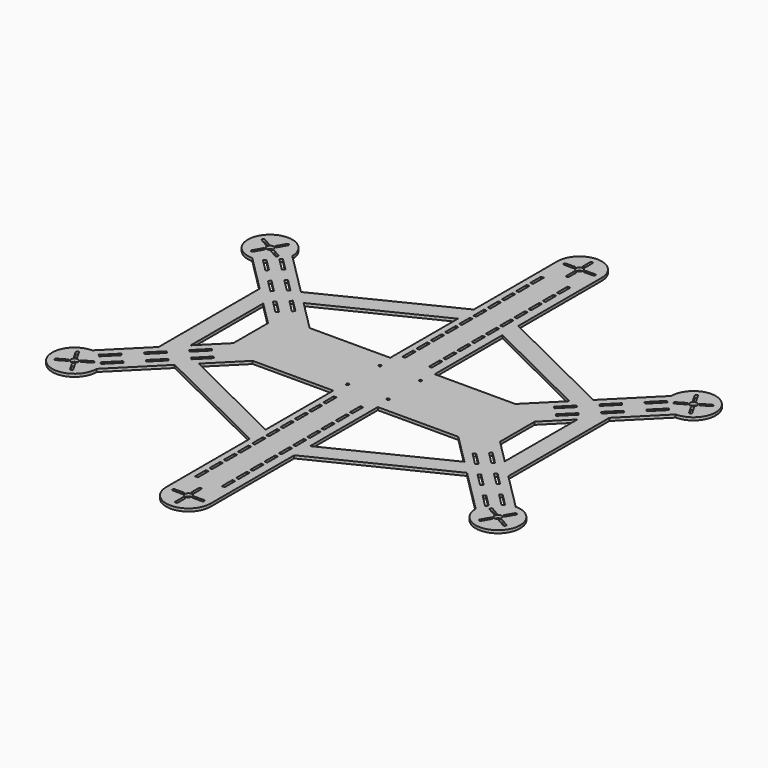
from build123d import *

# Parameters (mm, degrees)
F1_DEPTH  = 3.175
F2_W      = 3.175
F2_H      = 15
F3_DEPTH  = 25
F5_DEPTH  = 25
F6_DEPTH  = 3.175
F7_R      = 1.5
F8_DEPTH  = 25
F9_R      = 4
F9_W      = 3
F9_H      = 10
F9_W_2    = 10
F9_H_2    = 3
F10_DEPTH = 25


with BuildPart() as f1:
    # F0 (on Top) → F1 (new body)
    with BuildSketch(Plane.XY):
        with BuildLine():
            Line((-25, 275), (25, 275))
            ThreePointArc((25, 275), (0, 300), (-25, 275))
        make_face()
        with BuildLine():
            Line((25, 157.5), (25, 275))
            ThreePointArc((25, 275), (0, 250), (-25, 275))
            Line((-25, 275), (-25, 157.5))
            Line((-25, 157.5), (-25, 135.2001601372))
            Line((-25, 135.2001601372), (-25, 40))
            Line((-25, 40), (25, 40))
            Line((25, 40), (25, 135.2001601372))
            Line((25, 135.2001601372), (25, 157.5))
        make_face()
        with BuildLine():
            ThreePointArc((-25, 275), (0, 250), (25, 275))
            Line((25, 275), (-25, 275))
        make_face()
        Polygon((164.4069860407, 88.75), (25, 157.5), (25, 135.2001601372), (149.4723277158, 73.8153416751), align=None)
        Polygon((-25, 135.2001601372), (-25, 157.5), (-164.4069860407, 88.75), (-149.4723277158, 73.8153416751), align=None)
        with BuildLine():
            Line((213.1569860407, 137.5), (164.4069860407, 88.75))
            Line((164.4069860407, 88.75), (149.4723277158, 73.8153416751))
            Line((149.4723277158, 73.8153416751), (115.6569860407, 40))
            Line((115.6569860407, 40), (150, 40))
            Line((150, 40), (150, 24.3430139593))
            Line((150, 24.3430139593), (164.5977680896, 38.9407820489))
            Line((164.5977680896, 38.9407820489), (176.670305631, 51.0133195903))
            Line((176.670305631, 51.0133195903), (188.7428431724, 63.0858571317))
            Line((188.7428431724, 63.0858571317), (196.670305631, 71.0133195903))
            Line((196.670305631, 71.0133195903), (238.1569860407, 112.5))
            ThreePointArc((238.1569860407, 112.5), (220.4793165111, 119.8223304703), (213.1569860407, 137.5))
        make_face()
        with BuildLine():
            Line((-149.4723277158, 73.8153416751), (-164.4069860407, 88.75))
            Line((-164.4069860407, 88.75), (-213.1569860407, 137.5))
            ThreePointArc((-213.1569860407, 137.5), (-220.4793165111, 119.8223304703), (-238.1569860407, 112.5))
            Line((-238.1569860407, 112.5), (-196.670305631, 71.0133195903))
            Line((-196.670305631, 71.0133195903), (-188.7428431724, 63.0858571317))
            Line((-188.7428431724, 63.0858571317), (-176.670305631, 51.0133195903))
            Line((-176.670305631, 51.0133195903), (-164.5977680896, 38.9407820489))
            Line((-164.5977680896, 38.9407820489), (-150, 24.3430139593))
            Line((-150, 24.3430139593), (-150, 40))
            Line((-150, 40), (-115.6569860407, 40))
            Line((-115.6569860407, 40), (-149.4723277158, 73.8153416751))
        make_face()
        Polygon((115.6569860407, 40), (25, 40), (-25, 40), (-115.6569860407, 40), (-150, 40), (-150, 24.3430139593), (-150, -24.3430139593), (-150, -40), (-115.6569860407, -40), (-25, -40), (25, -40), (115.6569860407, -40), (150, -40), (150, -24.3430139593), (150, 24.3430139593), (150, 40), align=None)
        with BuildLine():
            ThreePointArc((263.1569860407, 137.5), (238.1569860407, 162.5), (213.1569860407, 137.5))
            ThreePointArc((213.1569860407, 137.5), (220.4793165111, 119.8223304703), (238.1569860407, 112.5))
            Line((238.1569860407, 112.5), (263.1569860407, 137.5))
        make_face()
        with BuildLine():
            ThreePointArc((-238.1569860407, 112.5), (-220.4793165111, 119.8223304703), (-213.1569860407, 137.5))
            ThreePointArc((-213.1569860407, 137.5), (-238.1569860407, 162.5), (-263.1569860407, 137.5))
            Line((-263.1569860407, 137.5), (-238.1569860407, 112.5))
        make_face()
        with BuildLine():
            ThreePointArc((238.1569860407, 112.5), (255.8346555704, 119.8223304703), (263.1569860407, 137.5))
            Line((263.1569860407, 137.5), (238.1569860407, 112.5))
        make_face()
        with BuildLine():
            Line((-238.1569860407, 112.5), (-263.1569860407, 137.5))
            ThreePointArc((-263.1569860407, 137.5), (-255.8346555704, 119.8223304703), (-238.1569860407, 112.5))
        make_face()
        Polygon((196.670305631, -71.0133195903), (196.670305631, 71.0133195903), (188.7428431724, 63.0858571317), (176.670305631, 51.0133195903), (176.670305631, -51.0133195903), align=None)
        Polygon((-188.7428431724, 63.0858571317), (-196.670305631, 71.0133195903), (-196.670305631, -71.0133195903), (-188.7428431724, -63.0858571317), (-176.670305631, -51.0133195903), (-176.670305631, 51.0133195903), align=None)
        with BuildLine():
            Line((238.1569860407, -112.5), (196.670305631, -71.0133195903))
            Line((196.670305631, -71.0133195903), (176.670305631, -51.0133195903))
            Line((176.670305631, -51.0133195903), (150, -24.3430139593))
            Line((150, -24.3430139593), (150, -40))
            Line((150, -40), (115.6569860407, -40))
            Line((115.6569860407, -40), (149.4723277158, -73.8153416751))
            Line((149.4723277158, -73.8153416751), (164.4069860407, -88.75))
            Line((164.4069860407, -88.75), (213.1569860407, -137.5))
            ThreePointArc((213.1569860407, -137.5), (220.4793165111, -119.8223304703), (238.1569860407, -112.5))
        make_face()
        with BuildLine():
            Line((-188.7428431724, -63.0858571317), (-196.670305631, -71.0133195903))
            Line((-196.670305631, -71.0133195903), (-238.1569860407, -112.5))
            ThreePointArc((-238.1569860407, -112.5), (-220.4793165111, -119.8223304703), (-213.1569860407, -137.5))
            Line((-213.1569860407, -137.5), (-164.4069860407, -88.75))
            Line((-164.4069860407, -88.75), (-149.4723277158, -73.8153416751))
            Line((-149.4723277158, -73.8153416751), (-115.6569860407, -40))
            Line((-115.6569860407, -40), (-150, -40))
            Line((-150, -40), (-150, -24.3430139593))
            Line((-150, -24.3430139593), (-164.5977680896, -38.9407820489))
            Line((-164.5977680896, -38.9407820489), (-176.670305631, -51.0133195903))
            Line((-176.670305631, -51.0133195903), (-188.7428431724, -63.0858571317))
        make_face()
        with BuildLine():
            Line((263.1569860407, -137.5), (238.1569860407, -112.5))
            ThreePointArc((238.1569860407, -112.5), (220.4793165111, -119.8223304703), (213.1569860407, -137.5))
            ThreePointArc((213.1569860407, -137.5), (238.1569860407, -162.5), (263.1569860407, -137.5))
        make_face()
        with BuildLine():
            ThreePointArc((263.1569860407, -137.5), (255.8346555704, -119.8223304703), (238.1569860407, -112.5))
            Line((238.1569860407, -112.5), (263.1569860407, -137.5))
        make_face()
        with BuildLine():
            Line((-263.1569860407, -137.5), (-238.1569860407, -112.5))
            ThreePointArc((-238.1569860407, -112.5), (-255.8346555704, -119.8223304703), (-263.1569860407, -137.5))
        make_face()
        with BuildLine():
            ThreePointArc((-213.1569860407, -137.5), (-220.4793165111, -119.8223304703), (-238.1569860407, -112.5))
            Line((-238.1569860407, -112.5), (-263.1569860407, -137.5))
            ThreePointArc((-263.1569860407, -137.5), (-238.1569860407, -162.5), (-213.1569860407, -137.5))
        make_face()
        Polygon((25, -157.5), (164.4069860407, -88.75), (149.4723277158, -73.8153416751), (25, -135.2001601372), align=None)
        Polygon((-149.4723277158, -73.8153416751), (-164.4069860407, -88.75), (-25, -157.5), (-25, -135.2001601372), align=None)
        with BuildLine():
            Line((25, -135.2001601372), (25, -40))
            Line((25, -40), (-25, -40))
            Line((-25, -40), (-25, -135.2001601372))
            Line((-25, -135.2001601372), (-25, -157.5))
            Line((-25, -157.5), (-25, -275))
            ThreePointArc((-25, -275), (0, -250), (25, -275))
            Line((25, -275), (25, -157.5))
            Line((25, -157.5), (25, -135.2001601372))
        make_face()
        with BuildLine():
            ThreePointArc((-25, -275), (0, -300), (25, -275))
            ThreePointArc((25, -275), (0, -250), (-25, -275))
        make_face()
    extrude(amount=F1_DEPTH)

    # F2 (on face) → F3 (cut)
    with BuildSketch(Plane.XY.offset(3.175)):
        with Locations((-16.3512844592, 235.6171465556)):
            Rectangle(F2_W, F2_H)
        with Locations((13.6487155408, 235.6171465556)):
            Rectangle(F2_W, F2_H)
        with Locations((-16.3512844592, 215.6171465556)):
            Rectangle(F2_W, F2_H)
        with Locations((13.6487155408, 215.6171465556)):
            Rectangle(F2_W, F2_H)
        with Locations((-16.3512844592, 195.6171465556)):
            Rectangle(F2_W, F2_H)
        with Locations((13.6487155408, 195.6171465556)):
            Rectangle(F2_W, F2_H)
        with Locations((-16.3512844592, 175.6171465556)):
            Rectangle(F2_W, F2_H)
        with Locations((13.6487155408, 175.6171465556)):
            Rectangle(F2_W, F2_H)
        with Locations((-16.3512844592, 155.6171465556)):
            Rectangle(F2_W, F2_H)
        with Locations((13.6487155408, 155.6171465556)):
            Rectangle(F2_W, F2_H)
        with Locations((-16.3512844592, 135.6171465556)):
            Rectangle(F2_W, F2_H)
        with Locations((13.6487155408, 135.6171465556)):
            Rectangle(F2_W, F2_H)
        with Locations((-16.3512844592, 115.6171465556)):
            Rectangle(F2_W, F2_H)
        with Locations((13.6487155408, 115.6171465556)):
            Rectangle(F2_W, F2_H)
        with Locations((-16.3512844592, 95.6171465556)):
            Rectangle(F2_W, F2_H)
        with Locations((13.6487155408, 95.6171465556)):
            Rectangle(F2_W, F2_H)
        with Locations((-16.3512844592, -235.6171465556)):
            Rectangle(F2_W, F2_H)
        with Locations((-16.3512844592, -215.6171465556)):
            Rectangle(F2_W, F2_H)
        with Locations((13.6487155408, -215.6171465556)):
            Rectangle(F2_W, F2_H)
        with Locations((13.6487155408, -115.6171465556)):
            Rectangle(F2_W, F2_H)
        with Locations((-16.3512844592, -115.6171465556)):
            Rectangle(F2_W, F2_H)
        with Locations((13.6487155408, -235.6171465556)):
            Rectangle(F2_W, F2_H)
        with Locations((-16.3512844592, -175.6171465556)):
            Rectangle(F2_W, F2_H)
        with Locations((13.6487155408, -95.6171465556)):
            Rectangle(F2_W, F2_H)
        with Locations((-16.3512844592, -155.6171465556)):
            Rectangle(F2_W, F2_H)
        with Locations((-16.3512844592, -135.6171465556)):
            Rectangle(F2_W, F2_H)
        with Locations((-16.3512844592, -95.6171465556)):
            Rectangle(F2_W, F2_H)
        with Locations((13.6487155408, -175.6171465556)):
            Rectangle(F2_W, F2_H)
        with Locations((13.6487155408, -195.6171465556)):
            Rectangle(F2_W, F2_H)
        with Locations((-16.3512844592, -195.6171465556)):
            Rectangle(F2_W, F2_H)
        with Locations((13.6487155408, -135.6171465556)):
            Rectangle(F2_W, F2_H)
        with Locations((13.6487155408, -155.6171465556)):
            Rectangle(F2_W, F2_H)
        with Locations((-16.3512844592, 75.6171465556)):
            Rectangle(F2_W, F2_H)
        with Locations((13.6487155408, 75.6171465556)):
            Rectangle(F2_W, F2_H)
        with Locations((-16.3512844592, 55.6171465556)):
            Rectangle(F2_W, F2_H)
        with Locations((13.6487155408, 55.6171465556)):
            Rectangle(F2_W, F2_H)
        with Locations((13.6487155408, -75.6171465556)):
            Rectangle(F2_W, F2_H)
        with Locations((-16.3512844592, -75.6171465556)):
            Rectangle(F2_W, F2_H)
        with Locations((13.6487155408, -55.6171465556)):
            Rectangle(F2_W, F2_H)
        with Locations((-16.3512844592, -55.6171465556)):
            Rectangle(F2_W, F2_H)
    extrude(amount=-F3_DEPTH, mode=Mode.SUBTRACT)

    # F4 (on face) → F5 (cut)
    with BuildSketch(Plane.XY.offset(3.175)):
        Polygon((-204.2056822111, 111.5586879855), (-201.9606181809, 113.8037520157), (-216.1027538046, 127.9458876395), (-218.3478178349, 125.7008236092), align=None)
        Polygon((-216.1027538046, -127.9458876395), (-201.9606181809, -113.8037520157), (-204.2056822111, -111.5586879855), (-218.3478178349, -125.7008236092), align=None)
        Polygon((-175.9214109637, 83.274416738), (-173.6763469334, 85.5194807683), (-187.8184825571, 99.661616392), (-190.0635465874, 97.4165523617), align=None)
        Polygon((-147.6371397162, 54.9901454905), (-145.3920756859, 57.2352095208), (-159.5342113097, 71.3773451445), (-161.7792753399, 69.1322811143), align=None)
        Polygon((-187.8184825571, -99.661616392), (-173.6763469334, -85.5194807683), (-175.9214109637, -83.274416738), (-190.0635465874, -97.4165523617), align=None)
        Polygon((-159.5342113097, -71.3773451445), (-145.3920756859, -57.2352095208), (-147.6371397162, -54.9901454905), (-161.7792753399, -69.1322811143), align=None)
        Polygon((-228.602633929, 115.446007515), (-214.4604983053, 101.3038718913), (-212.215434275, 103.5489359216), (-226.3575698988, 117.6910715453), align=None)
        Polygon((-200.3183626816, 87.1617362676), (-186.1762270578, 73.0196006438), (-183.9311630276, 75.2646646741), (-198.0732986513, 89.4068002978), align=None)
        Polygon((-169.7890274038, 61.1225290504), (-172.0340914341, 58.8774650201), (-157.8919558104, 44.7353293964), (-155.6468917801, 46.9803934266), align=None)
        Polygon((-183.9311630276, -75.2646646741), (-186.1762270578, -73.0196006438), (-200.3183626816, -87.1617362676), (-198.0732986513, -89.4068002978), align=None)
        Polygon((-212.215434275, -103.5489359216), (-214.4604983053, -101.3038718913), (-228.602633929, -115.446007515), (-226.3575698988, -117.6910715453), align=None)
        Polygon((-157.8919558104, -44.7353293964), (-172.0340914341, -58.8774650201), (-169.7890274038, -61.1225290504), (-155.6468917801, -46.9803934266), align=None)
        Polygon((145.3920756859, -57.2352095208), (159.5342113097, -71.3773451445), (161.7792753399, -69.1322811143), (147.6371397162, -54.9901454905), align=None)
        Polygon((175.9214109637, -83.274416738), (173.6763469334, -85.5194807683), (187.8184825571, -99.661616392), (190.0635465874, -97.4165523617), align=None)
        Polygon((212.215434275, 103.5489359216), (214.4604983053, 101.3038718913), (228.602633929, 115.446007515), (226.3575698988, 117.6910715453), align=None)
        Polygon((187.8184825571, 99.661616392), (173.6763469334, 85.5194807683), (175.9214109637, 83.274416738), (190.0635465874, 97.4165523617), align=None)
        Polygon((218.3478178349, 125.7008236092), (216.1027538046, 127.9458876395), (201.9606181809, 113.8037520157), (204.2056822111, 111.5586879855), align=None)
        Polygon((161.7792753399, 69.1322811143), (159.5342113097, 71.3773451445), (145.3920756859, 57.2352095208), (147.6371397162, 54.9901454905), align=None)
        Polygon((198.0732986513, -89.4068002978), (200.3183626816, -87.1617362676), (186.1762270578, -73.0196006438), (183.9311630276, -75.2646646741), align=None)
        Polygon((183.9311630276, 75.2646646741), (186.1762270578, 73.0196006438), (200.3183626816, 87.1617362676), (198.0732986513, 89.4068002978), align=None)
        Polygon((169.7890274038, -61.1225290504), (172.0340914341, -58.8774650201), (157.8919558104, -44.7353293964), (155.6468917801, -46.9803934266), align=None)
        Polygon((157.8919558104, 44.7353293964), (172.0340914341, 58.8774650201), (169.7890274038, 61.1225290504), (155.6468917801, 46.9803934266), align=None)
        Polygon((228.602633929, -115.446007515), (214.4604983053, -101.3038718913), (212.215434275, -103.5489359216), (226.3575698988, -117.6910715453), align=None)
        Polygon((218.3478178349, -125.7008236092), (204.2056822111, -111.5586879855), (201.9606181809, -113.8037520157), (216.1027538046, -127.9458876395), align=None)
    extrude(amount=-F5_DEPTH, mode=Mode.SUBTRACT)

    # F2 (on face) → F6 (cut)
    with BuildSketch(Plane.XY.offset(3.175)):
        with Locations((-16.3512844592, 235.6171465556)):
            Rectangle(F2_W, F2_H)
        with Locations((13.6487155408, 235.6171465556)):
            Rectangle(F2_W, F2_H)
        with Locations((-16.3512844592, 215.6171465556)):
            Rectangle(F2_W, F2_H)
        with Locations((13.6487155408, 215.6171465556)):
            Rectangle(F2_W, F2_H)
        with Locations((-16.3512844592, 195.6171465556)):
            Rectangle(F2_W, F2_H)
        with Locations((13.6487155408, 195.6171465556)):
            Rectangle(F2_W, F2_H)
        with Locations((-16.3512844592, 175.6171465556)):
            Rectangle(F2_W, F2_H)
        with Locations((13.6487155408, 175.6171465556)):
            Rectangle(F2_W, F2_H)
        with Locations((-16.3512844592, 155.6171465556)):
            Rectangle(F2_W, F2_H)
        with Locations((13.6487155408, 155.6171465556)):
            Rectangle(F2_W, F2_H)
        with Locations((-16.3512844592, 135.6171465556)):
            Rectangle(F2_W, F2_H)
        with Locations((13.6487155408, 135.6171465556)):
            Rectangle(F2_W, F2_H)
        with Locations((-16.3512844592, 115.6171465556)):
            Rectangle(F2_W, F2_H)
        with Locations((13.6487155408, 115.6171465556)):
            Rectangle(F2_W, F2_H)
        with Locations((-16.3512844592, 95.6171465556)):
            Rectangle(F2_W, F2_H)
        with Locations((13.6487155408, 95.6171465556)):
            Rectangle(F2_W, F2_H)
        with Locations((-16.3512844592, -235.6171465556)):
            Rectangle(F2_W, F2_H)
        with Locations((-16.3512844592, -215.6171465556)):
            Rectangle(F2_W, F2_H)
        with Locations((13.6487155408, -215.6171465556)):
            Rectangle(F2_W, F2_H)
        with Locations((13.6487155408, -115.6171465556)):
            Rectangle(F2_W, F2_H)
        with Locations((-16.3512844592, -115.6171465556)):
            Rectangle(F2_W, F2_H)
        with Locations((13.6487155408, -235.6171465556)):
            Rectangle(F2_W, F2_H)
        with Locations((-16.3512844592, -175.6171465556)):
            Rectangle(F2_W, F2_H)
        with Locations((13.6487155408, -95.6171465556)):
            Rectangle(F2_W, F2_H)
        with Locations((-16.3512844592, -155.6171465556)):
            Rectangle(F2_W, F2_H)
        with Locations((-16.3512844592, -135.6171465556)):
            Rectangle(F2_W, F2_H)
        with Locations((-16.3512844592, -95.6171465556)):
            Rectangle(F2_W, F2_H)
        with Locations((13.6487155408, -175.6171465556)):
            Rectangle(F2_W, F2_H)
        with Locations((13.6487155408, -195.6171465556)):
            Rectangle(F2_W, F2_H)
        with Locations((-16.3512844592, -195.6171465556)):
            Rectangle(F2_W, F2_H)
        with Locations((13.6487155408, -135.6171465556)):
            Rectangle(F2_W, F2_H)
        with Locations((13.6487155408, -155.6171465556)):
            Rectangle(F2_W, F2_H)
        with Locations((-16.3512844592, 75.6171465556)):
            Rectangle(F2_W, F2_H)
        with Locations((13.6487155408, 75.6171465556)):
            Rectangle(F2_W, F2_H)
        with Locations((-16.3512844592, 55.6171465556)):
            Rectangle(F2_W, F2_H)
        with Locations((13.6487155408, 55.6171465556)):
            Rectangle(F2_W, F2_H)
        with Locations((13.6487155408, -75.6171465556)):
            Rectangle(F2_W, F2_H)
        with Locations((-16.3512844592, -75.6171465556)):
            Rectangle(F2_W, F2_H)
        with Locations((13.6487155408, -55.6171465556)):
            Rectangle(F2_W, F2_H)
        with Locations((-16.3512844592, -55.6171465556)):
            Rectangle(F2_W, F2_H)
    extrude(amount=-F6_DEPTH, mode=Mode.SUBTRACT)

    # F7 (on face) → F8 (cut)
    with BuildSketch(Plane.XY.offset(3.175)):
        with Locations((-22.772, 22.772)):
            Circle(F7_R)
        with Locations((22.772, 22.772)):
            Circle(F7_R)
        with Locations((22.772, -22.772)):
            Circle(F7_R)
        with Locations((-22.772, -22.772)):
            Circle(F7_R)
    extrude(amount=-F8_DEPTH, mode=Mode.SUBTRACT)

    # F9 (on face) → F10 (cut)
    with BuildSketch(Plane.XY.offset(3.175)):
        with Locations((0, 275)):
            Circle(F9_R)
        with BuildLine():
            ThreePointArc((-1.5, 281.3555584285), (0, 279.8555584285), (1.5, 281.3555584285))
            Line((1.5, 281.3555584285), (-1.5, 281.3555584285))
        make_face()
        with Locations((0, 286.3555584285)):
            Rectangle(F9_W, F9_H)
        with BuildLine():
            Line((-1.5, 291.3555584285), (1.5, 291.3555584285))
            ThreePointArc((1.5, 291.3555584285), (0, 292.8555584285), (-1.5, 291.3555584285))
        make_face()
        with BuildLine():
            ThreePointArc((-6.3555584285, 273.5), (-4.8555584285, 275), (-6.3555584285, 276.5))
            Line((-6.3555584285, 276.5), (-6.3555584285, 273.5))
        make_face()
        with Locations((-11.3555584285, 275)):
            Rectangle(F9_W_2, F9_H_2)
        with BuildLine():
            Line((-16.3555584285, 273.5), (-16.3555584285, 276.5))
            ThreePointArc((-16.3555584285, 276.5), (-17.8555584285, 275), (-16.3555584285, 273.5))
        make_face()
        with BuildLine():
            ThreePointArc((1.5, 268.6444415715), (0, 270.1444415715), (-1.5, 268.6444415715))
            Line((-1.5, 268.6444415715), (1.5, 268.6444415715))
        make_face()
        with Locations((0, 263.6444415715)):
            Rectangle(F9_W, F9_H)
        with BuildLine():
            Line((1.5, 258.6444415715), (-1.5, 258.6444415715))
            ThreePointArc((-1.5, 258.6444415715), (0, 257.1444415715), (1.5, 258.6444415715))
        make_face()
        with BuildLine():
            ThreePointArc((6.3555584285, 276.5), (4.8555584285, 275), (6.3555584285, 273.5))
            Line((6.3555584285, 273.5), (6.3555584285, 276.5))
        make_face()
        with Locations((11.3555584285, 275)):
            Rectangle(F9_W_2, F9_H_2)
        with BuildLine():
            Line((16.3555584285, 276.5), (16.3555584285, 273.5))
            ThreePointArc((16.3555584285, 273.5), (17.8555584285, 275), (16.3555584285, 276.5))
        make_face()
        Polygon((-231.8949388808, 135.6165043144), (-233.3949388808, 133.018428103), (-224.7346848429, 128.018428103), (-223.2346848429, 130.6165043144), align=None)
        with BuildLine():
            ThreePointArc((-231.8949388808, 135.6165043144), (-233.9439769865, 135.0674662087), (-233.3949388808, 133.018428103))
            Line((-233.3949388808, 133.018428103), (-231.8949388808, 135.6165043144))
        make_face()
        with BuildLine():
            Line((-223.2346848429, 130.6165043144), (-224.7346848429, 128.018428103))
            ThreePointArc((-224.7346848429, 128.018428103), (-222.6856467373, 128.5674662087), (-223.2346848429, 130.6165043144))
        make_face()
        with BuildLine():
            Line((-231.2702728265, 152.4095745151), (-228.6721966152, 150.9095745151))
            ThreePointArc((-228.6721966152, 150.9095745151), (-229.2212347209, 152.9586126208), (-231.2702728265, 152.4095745151))
        make_face()
        Polygon((-233.6721966152, 142.2493204773), (-228.6721966152, 150.9095745151), (-231.2702728265, 152.4095745151), (-236.2702728265, 143.7493204773), align=None)
        with BuildLine():
            ThreePointArc((-236.2702728265, 143.7493204773), (-235.7212347209, 141.7002823716), (-233.6721966152, 142.2493204773))
            Line((-233.6721966152, 142.2493204773), (-236.2702728265, 143.7493204773))
        make_face()
        with BuildLine():
            Line((-245.0277550437, 122.5809163308), (-247.6258312551, 124.0809163308))
            ThreePointArc((-247.6258312551, 124.0809163308), (-247.0767931494, 122.0318782251), (-245.0277550437, 122.5809163308))
        make_face()
        Polygon((-242.6258312551, 132.7411703686), (-247.6258312551, 124.0809163308), (-245.0277550437, 122.5809163308), (-240.0277550437, 131.2411703686), align=None)
        with BuildLine():
            ThreePointArc((-240.0277550437, 131.2411703686), (-240.5767931494, 133.2902084743), (-242.6258312551, 132.7411703686))
            Line((-242.6258312551, 132.7411703686), (-240.0277550437, 131.2411703686))
        make_face()
        with BuildLine():
            Line((-253.0633430273, 144.3739865315), (-251.5633430273, 146.9720627429))
            ThreePointArc((-251.5633430273, 146.9720627429), (-253.612381133, 146.4230246372), (-253.0633430273, 144.3739865315))
        make_face()
        Polygon((-242.9030889895, 141.9720627429), (-251.5633430273, 146.9720627429), (-253.0633430273, 144.3739865315), (-244.4030889895, 139.3739865315), align=None)
        with BuildLine():
            ThreePointArc((-244.4030889895, 139.3739865315), (-242.3540508838, 139.9230246372), (-242.9030889895, 141.9720627429))
            Line((-242.9030889895, 141.9720627429), (-244.4030889895, 139.3739865315))
        make_face()
        with Locations((-238.1490139351, 137.4952454229)):
            Circle(F9_R)
        Polygon((-233.3868352435, -133.0234104997), (-231.8868352435, -135.621486711), (-223.2265812056, -130.621486711), (-224.7265812056, -128.0234104997), align=None)
        with BuildLine():
            ThreePointArc((-233.3868352435, -133.0234104997), (-233.9358733492, -135.0724486054), (-231.8868352435, -135.621486711))
            Line((-231.8868352435, -135.621486711), (-233.3868352435, -133.0234104997))
        make_face()
        with BuildLine():
            Line((-224.7265812056, -128.0234104997), (-223.2265812056, -130.621486711))
            ThreePointArc((-223.2265812056, -130.621486711), (-222.6775431, -128.5724486054), (-224.7265812056, -128.0234104997))
        make_face()
        with BuildLine():
            Line((-247.6177276178, -124.0858987274), (-245.0196514064, -122.5858987274))
            ThreePointArc((-245.0196514064, -122.5858987274), (-247.0686895121, -122.0368606218), (-247.6177276178, -124.0858987274))
        make_face()
        Polygon((-240.0196514064, -131.2461527653), (-245.0196514064, -122.5858987274), (-247.6177276178, -124.0858987274), (-242.6177276178, -132.7461527653), align=None)
        with BuildLine():
            ThreePointArc((-242.6177276178, -132.7461527653), (-240.5686895121, -133.2951908709), (-240.0196514064, -131.2461527653))
            Line((-240.0196514064, -131.2461527653), (-242.6177276178, -132.7461527653))
        make_face()
        with BuildLine():
            Line((-228.6640929779, -150.9145569118), (-231.2621691892, -152.4145569118))
            ThreePointArc((-231.2621691892, -152.4145569118), (-229.2131310836, -152.9635950175), (-228.6640929779, -150.9145569118))
        make_face()
        Polygon((-236.2621691892, -143.754302874), (-231.2621691892, -152.4145569118), (-228.6640929779, -150.9145569118), (-233.6640929779, -142.254302874), align=None)
        with BuildLine():
            ThreePointArc((-233.6640929779, -142.254302874), (-235.7131310836, -141.7052647683), (-236.2621691892, -143.754302874))
            Line((-236.2621691892, -143.754302874), (-233.6640929779, -142.254302874))
        make_face()
        with BuildLine():
            Line((-251.55523939, -146.9770451396), (-253.05523939, -144.3789689282))
            ThreePointArc((-253.05523939, -144.3789689282), (-253.6042774957, -146.4280070339), (-251.55523939, -146.9770451396))
        make_face()
        Polygon((-244.3949853522, -139.3789689282), (-253.05523939, -144.3789689282), (-251.55523939, -146.9770451396), (-242.8949853522, -141.9770451396), align=None)
        with BuildLine():
            ThreePointArc((-242.8949853522, -141.9770451396), (-242.3459472465, -139.9280070339), (-244.3949853522, -139.3789689282))
            Line((-244.3949853522, -139.3789689282), (-242.8949853522, -141.9770451396))
        make_face()
        with Locations((-238.1409102978, -137.5002278196)):
            Circle(F9_R)
        with Locations((0.0162072746, -263.6353880566)):
            Rectangle(F9_W, F9_H)
        with BuildLine():
            ThreePointArc((-1.4837927254, -268.6353880566), (0.0162072746, -270.1353880566), (1.5162072746, -268.6353880566))
            Line((1.5162072746, -268.6353880566), (-1.4837927254, -268.6353880566))
        make_face()
        with BuildLine():
            Line((-1.4837927254, -258.6353880566), (1.5162072746, -258.6353880566))
            ThreePointArc((1.5162072746, -258.6353880566), (0.0162072746, -257.1353880566), (-1.4837927254, -258.6353880566))
        make_face()
        with BuildLine():
            Line((-16.3393511539, -276.4909464851), (-16.3393511539, -273.4909464851))
            ThreePointArc((-16.3393511539, -273.4909464851), (-17.8393511539, -274.9909464851), (-16.3393511539, -276.4909464851))
        make_face()
        with Locations((-11.3393511539, -274.9909464851)):
            Rectangle(F9_W_2, F9_H_2)
        with BuildLine():
            ThreePointArc((-6.3393511539, -276.4909464851), (-4.8393511539, -274.9909464851), (-6.3393511539, -273.4909464851))
            Line((-6.3393511539, -273.4909464851), (-6.3393511539, -276.4909464851))
        make_face()
        with BuildLine():
            Line((16.3717657032, -273.4909464851), (16.3717657032, -276.4909464851))
            ThreePointArc((16.3717657032, -276.4909464851), (17.8717657032, -274.9909464851), (16.3717657032, -273.4909464851))
        make_face()
        with Locations((11.3717657032, -274.9909464851)):
            Rectangle(F9_W_2, F9_H_2)
        with BuildLine():
            ThreePointArc((6.3717657032, -273.4909464851), (4.8717657032, -274.9909464851), (6.3717657032, -276.4909464851))
            Line((6.3717657032, -276.4909464851), (6.3717657032, -273.4909464851))
        make_face()
        with BuildLine():
            Line((1.5162072746, -291.3465049137), (-1.4837927254, -291.3465049137))
            ThreePointArc((-1.4837927254, -291.3465049137), (0.0162072746, -292.8465049137), (1.5162072746, -291.3465049137))
        make_face()
        with Locations((0.0162072746, -286.3465049137)):
            Rectangle(F9_W, F9_H)
        with BuildLine():
            ThreePointArc((1.5162072746, -281.3465049137), (0.0162072746, -279.8465049137), (-1.4837927254, -281.3465049137))
            Line((-1.4837927254, -281.3465049137), (1.5162072746, -281.3465049137))
        make_face()
        with Locations((0.0162072746, -274.9909464851)):
            Circle(F9_R)
        Polygon((231.9111461554, -135.6074507995), (233.4111461554, -133.0093745881), (224.7508921176, -128.0093745881), (223.2508921176, -130.6074507995), align=None)
        with BuildLine():
            ThreePointArc((231.9111461554, -135.6074507995), (233.9601842611, -135.0584126938), (233.4111461554, -133.0093745881))
            Line((233.4111461554, -133.0093745881), (231.9111461554, -135.6074507995))
        make_face()
        with BuildLine():
            Line((223.2508921176, -130.6074507995), (224.7508921176, -128.0093745881))
            ThreePointArc((224.7508921176, -128.0093745881), (222.7018540119, -128.5584126938), (223.2508921176, -130.6074507995))
        make_face()
        with BuildLine():
            Line((231.2864801012, -152.4005210003), (228.6884038898, -150.9005210003))
            ThreePointArc((228.6884038898, -150.9005210003), (229.2374419955, -152.9495591059), (231.2864801012, -152.4005210003))
        make_face()
        Polygon((233.6884038898, -142.2402669624), (228.6884038898, -150.9005210003), (231.2864801012, -152.4005210003), (236.2864801012, -143.7402669624), align=None)
        with BuildLine():
            ThreePointArc((236.2864801012, -143.7402669624), (235.7374419955, -141.6912288568), (233.6884038898, -142.2402669624))
            Line((233.6884038898, -142.2402669624), (236.2864801012, -143.7402669624))
        make_face()
        with BuildLine():
            Line((245.0439623183, -122.5718628159), (247.6420385297, -124.0718628159))
            ThreePointArc((247.6420385297, -124.0718628159), (247.093000424, -122.0228247102), (245.0439623183, -122.5718628159))
        make_face()
        Polygon((242.6420385297, -132.7321168537), (247.6420385297, -124.0718628159), (245.0439623183, -122.5718628159), (240.0439623183, -131.2321168537), align=None)
        with BuildLine():
            ThreePointArc((240.0439623183, -131.2321168537), (240.593000424, -133.2811549594), (242.6420385297, -132.7321168537))
            Line((242.6420385297, -132.7321168537), (240.0439623183, -131.2321168537))
        make_face()
        with BuildLine():
            Line((253.0795503019, -144.3649330167), (251.5795503019, -146.963009228))
            ThreePointArc((251.5795503019, -146.963009228), (253.6285884076, -146.4139711223), (253.0795503019, -144.3649330167))
        make_face()
        Polygon((242.9192962641, -141.963009228), (251.5795503019, -146.963009228), (253.0795503019, -144.3649330167), (244.4192962641, -139.3649330167), align=None)
        with BuildLine():
            ThreePointArc((244.4192962641, -139.3649330167), (242.3702581584, -139.9139711223), (242.9192962641, -141.963009228))
            Line((242.9192962641, -141.963009228), (244.4192962641, -139.3649330167))
        make_face()
        with Locations((238.1652212097, -137.4861919081)):
            Circle(F9_R)
        Polygon((233.4030425181, 133.0324640145), (231.9030425181, 135.6305402259), (223.2427884802, 130.6305402259), (224.7427884802, 128.0324640145), align=None)
        with BuildLine():
            ThreePointArc((233.4030425181, 133.0324640145), (233.9520806238, 135.0815021202), (231.9030425181, 135.6305402259))
            Line((231.9030425181, 135.6305402259), (233.4030425181, 133.0324640145))
        make_face()
        with BuildLine():
            Line((224.7427884802, 128.0324640145), (223.2427884802, 130.6305402259))
            ThreePointArc((223.2427884802, 130.6305402259), (222.6937503746, 128.5815021202), (224.7427884802, 128.0324640145))
        make_face()
        with BuildLine():
            Line((247.6339348924, 124.0949522423), (245.035858681, 122.5949522423))
            ThreePointArc((245.035858681, 122.5949522423), (247.0848967867, 122.0459141366), (247.6339348924, 124.0949522423))
        make_face()
        Polygon((240.035858681, 131.2552062801), (245.035858681, 122.5949522423), (247.6339348924, 124.0949522423), (242.6339348924, 132.7552062801), align=None)
        with BuildLine():
            ThreePointArc((242.6339348924, 132.7552062801), (240.5848967867, 133.3042443858), (240.035858681, 131.2552062801))
            Line((240.035858681, 131.2552062801), (242.6339348924, 132.7552062801))
        make_face()
        with BuildLine():
            Line((228.6803002525, 150.9236104267), (231.2783764638, 152.4236104267))
            ThreePointArc((231.2783764638, 152.4236104267), (229.2293383582, 152.9726485324), (228.6803002525, 150.9236104267))
        make_face()
        Polygon((236.2783764638, 143.7633563888), (231.2783764638, 152.4236104267), (228.6803002525, 150.9236104267), (233.6803002525, 142.2633563888), align=None)
        with BuildLine():
            ThreePointArc((233.6803002525, 142.2633563888), (235.7293383582, 141.7143182832), (236.2783764638, 143.7633563888))
            Line((236.2783764638, 143.7633563888), (233.6803002525, 142.2633563888))
        make_face()
        with BuildLine():
            Line((251.5714466646, 146.9860986544), (253.0714466646, 144.3880224431))
            ThreePointArc((253.0714466646, 144.3880224431), (253.6204847703, 146.4370605488), (251.5714466646, 146.9860986544))
        make_face()
        Polygon((244.4111926268, 139.3880224431), (253.0714466646, 144.3880224431), (251.5714466646, 146.9860986544), (242.9111926268, 141.9860986544), align=None)
        with BuildLine():
            ThreePointArc((242.9111926268, 141.9860986544), (242.3621545211, 139.9370605488), (244.4111926268, 139.3880224431))
            Line((244.4111926268, 139.3880224431), (242.9111926268, 141.9860986544))
        make_face()
        with Locations((238.1571175724, 137.5092813345)):
            Circle(F9_R)
    extrude(amount=-F10_DEPTH, mode=Mode.SUBTRACT)


solid = f1.part
